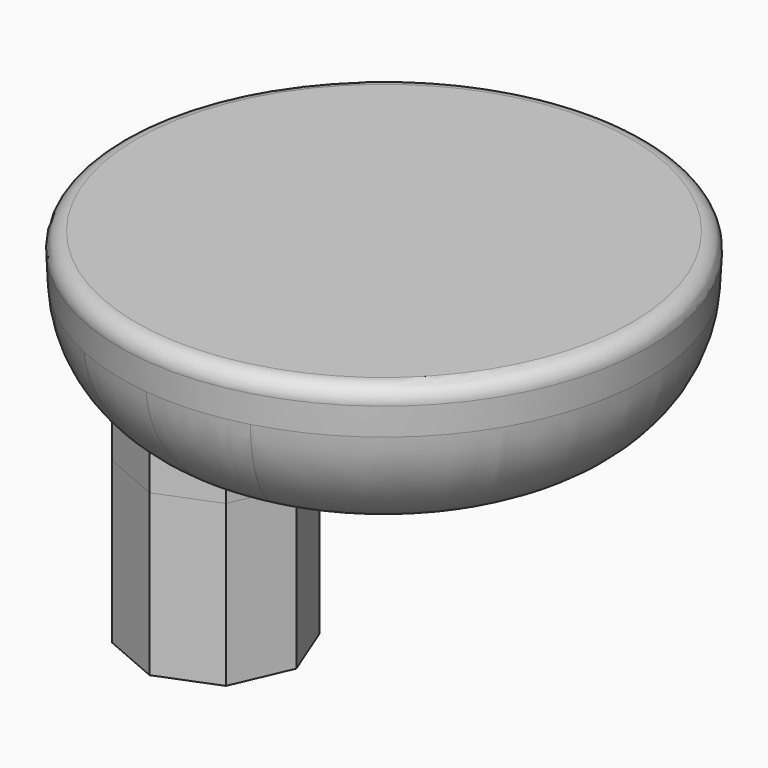
from build123d import *

# Parameters (mm, degrees)
F0_R     = 40.5620134448
F1_DEPTH = 25.4
F1_TAPER = -3
F2_R     = 2.54
F4_DEPTH = 25.4


# Not quite as in the source:
# - a fillet or chamfer that OpenCascade refuses, or shapes differently, is made with other operations: its cross-section is extruded or revolved along the edge and cut away or added


with BuildPart() as f1:
    # F0 (on Top) → F1 (new body)
    with BuildSketch(Plane.XY):
        with Locations((-84.2179358006, 32.7308289707)):
            Circle(F0_R)
    extrude(amount=F1_DEPTH, taper=F1_TAPER)

    # F2
    f2_edges = [f1.edges().sort_by_distance(p)[0] for p in [
        (-126.111107, 32.730829, 25.4),
    ]]
    fillet(f2_edges, radius=F2_R)

    # F3 (on face) → F4 (join)
    with BuildSketch(Plane(origin=(0, 0, 0), x_dir=(1, 0, 0), z_dir=(0, 0, -1))):
        Polygon((-84.1343444512, -19.9111274666), (-80.4951596333, -10.7477918976), (-84.4013240897, -1.6950429158), (-93.5646596587, 1.9441419021), (-102.6174086406, -1.9620225542), (-106.2565934585, -11.1253581232), (-102.3504290021, -20.1781071051), (-93.1870934331, -23.817291923), align=None)
    extrude(amount=F4_DEPTH)

    # F5: fillet of radius 19.304 on 1 edges, made by hand


with BuildPart() as f5_tool1:
    # F5_s2 → F5_t3 (revolve)
    with BuildSketch(Plane.XZ.offset(-32.7308289707)):
        with BuildLine():
            ThreePointArc((-42.6971898128, 18.2937067007), (-48.6867376225, 5.301373142), (-61.9747343517, 0))
            Line((-61.9747343517, 0), (-43.6559223558, 0))
            Line((-43.6559223558, 0), (-42.6971898128, 18.2937067007))
        make_face()
    revolve(axis=Axis((-84.2179358006, 32.7308289707, 0), (0, 0, 1)))

    split(bisect_by=Plane(origin=(-65.841803323, -26.1488285825, 0), x_dir=(0, 0, 1), z_dir=(0.929388426, 0.3691031748, 0)), keep=Keep.TOP)


with BuildPart() as f5_tool5:
    # F5_s6 → F5_t7 (revolve)
    with BuildSketch(Plane.XZ.offset(-32.7308289707)):
        with BuildLine():
            ThreePointArc((-42.6971898128, 18.2937067007), (-48.6867376225, 5.301373142), (-61.9747343517, 0))
            Line((-61.9747343517, 0), (-43.6559223558, 0))
            Line((-43.6559223558, 0), (-42.6971898128, 18.2937067007))
        make_face()
    revolve(axis=Axis((-84.2179358006, 32.7308289707, 0), (0, 0, 1)))

    split(bisect_by=Plane(origin=(-71.7703043479, 30.9681194552, 0), x_dir=(0, 0, 1), z_dir=(0.9181722162, -0.3961815006, 0)), keep=Keep.TOP)


with BuildPart() as f5_tool9:
    # F5_s10 → F5_t11 (revolve)
    with BuildSketch(Plane.XZ.offset(-32.7308289707)):
        with BuildLine():
            ThreePointArc((-42.6971898128, 18.2937067007), (-48.6867376225, 5.301373142), (-61.9747343517, 0))
            Line((-61.9747343517, 0), (-43.6559223558, 0))
            Line((-43.6559223558, 0), (-42.6971898128, 18.2937067007))
        make_face()
    revolve(axis=Axis((-84.2179358006, 32.7308289707, 0), (0, 0, 1)))

    split(bisect_by=Plane(origin=(-93.6255737167, 40.3984346626, 0), x_dir=(0, 0, 1), z_dir=(-0.9181722162, 0.3961815006, 0)), keep=Keep.TOP)


with BuildPart() as f5_tool13:
    # F5_s14 → F5_t15 (revolve)
    with BuildSketch(Plane.XZ.offset(-32.7308289707)):
        with BuildLine():
            ThreePointArc((-42.6971898128, 18.2937067007), (-48.6867376225, 5.301373142), (-61.9747343517, 0))
            Line((-61.9747343517, 0), (-43.6559223558, 0))
            Line((-43.6559223558, 0), (-42.6971898128, 18.2937067007))
        make_face()
    revolve(axis=Axis((-84.2179358006, 32.7308289707, 0), (0, 0, 1)))

    split(bisect_by=Plane(origin=(-12.0800640476, 30.4171637609, 0), x_dir=(0, 0, 1), z_dir=(0.3691031748, -0.929388426, 0)), keep=Keep.TOP)


with BuildPart() as f5_tool17:
    # F5_s18 → F5_t19 (revolve)
    with BuildSketch(Plane.XZ.offset(-32.7308289707)):
        with BuildLine():
            ThreePointArc((-42.6971898128, 18.2937067007), (-48.6867376225, 5.301373142), (-61.9747343517, 0))
            Line((-61.9747343517, 0), (-43.6559223558, 0))
            Line((-43.6559223558, 0), (-42.6971898128, 18.2937067007))
        make_face()
    revolve(axis=Axis((-84.2179358006, 32.7308289707, 0), (0, 0, 1)))

    split(bisect_by=Plane(origin=(-15.3930951173, -35.6743367329, 0), x_dir=(0, 0, 1), z_dir=(-0.3961815006, -0.9181722162, 0)), keep=Keep.TOP)


with BuildPart() as f5_tool21:
    # F5_s22 → F5_t23 (revolve)
    with BuildSketch(Plane.XZ.offset(-32.7308289707)):
        with BuildLine():
            ThreePointArc((-42.6971898128, 18.2937067007), (-48.6867376225, 5.301373142), (-61.9747343517, 0))
            Line((-61.9747343517, 0), (-43.6559223558, 0))
            Line((-43.6559223558, 0), (-42.6971898128, 18.2937067007))
        make_face()
    revolve(axis=Axis((-84.2179358006, 32.7308289707, 0), (0, 0, 1)))

    split(bisect_by=Plane(origin=(-87.9640523303, -34.9345979258, 0), x_dir=(0, 0, 1), z_dir=(-0.929388426, -0.3691031748, 0)), keep=Keep.TOP)


with BuildPart() as f1_1:
    add(f1.part)

    # F5_t25: cut F5_tool1, F5_tool5, F5_tool9, F5_tool13, F5_tool17, F5_tool21
    add([f5_tool1.part, f5_tool5.part, f5_tool9.part, f5_tool13.part, f5_tool17.part, f5_tool21.part], mode=Mode.SUBTRACT)


solid = f1_1.part
